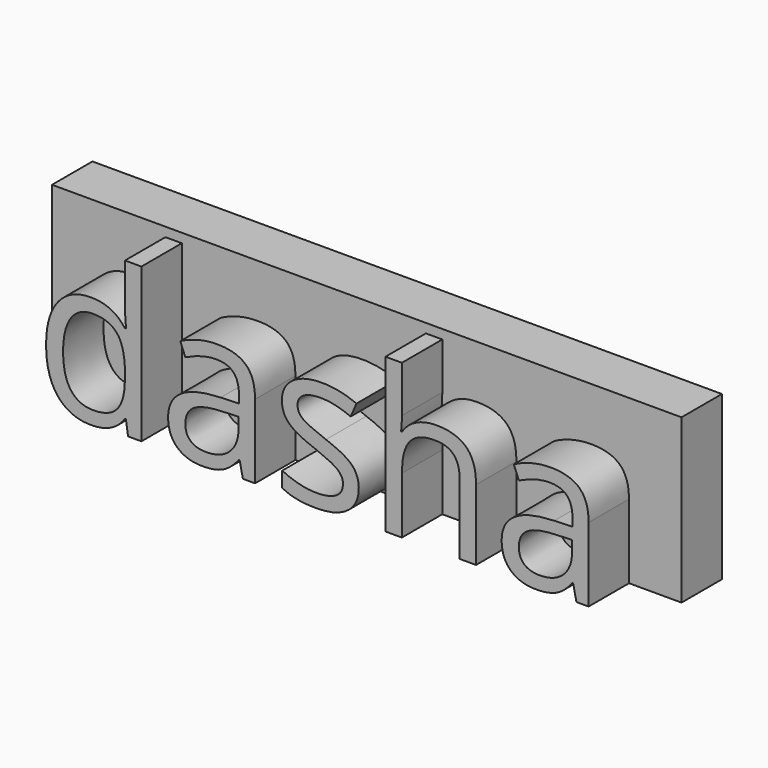
from build123d import *

# Parameters (mm, degrees)
F0_TEXT_SIZE = 20.0487763828
F1_DEPTH     = 5
F2_W         = 62.3139794916
F2_H         = 16.1501821131
F3_DEPTH     = 5


# Not quite as in the source:
# - Text() gives the source's letters only with a copy of the font that has no kerning and outlines rounded to 1/6400 em; it was checked with that copy


with BuildPart() as f1:
    # F0 (on Front) → F1 (new body)
    with BuildSketch(Plane.XZ):
        with Locations((-25.7259532809, 0)):
            Text('dasha', F0_TEXT_SIZE, font='Open Sans', text_align=(TextAlign.LEFT, TextAlign.BOTTOM))
    extrude(amount=F1_DEPTH)


with BuildPart() as f3:
    # F2 (on Front) → F3 (new body)
    with BuildSketch(Plane.XZ):
        with Locations((3.144283779, 8.0750910565)):
            Rectangle(F2_W, F2_H)
    extrude(amount=-F3_DEPTH)


solid = Compound([f1.part, f3.part])
